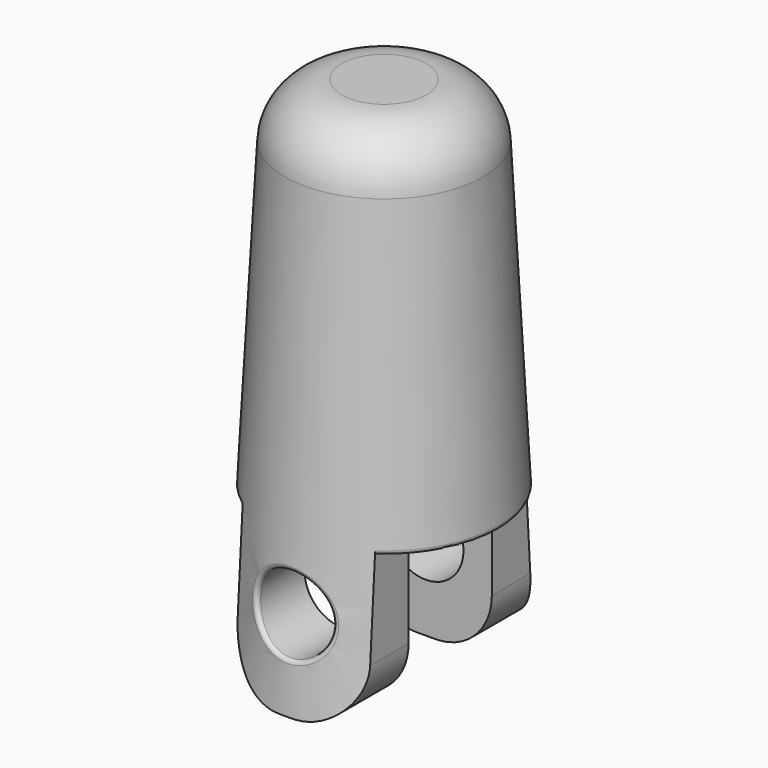
from build123d import *

# Parameters (mm, degrees)
F0_R          = 6.5
F1_DEPTH      = 27
F1_TAPER      = 3
F2_R          = 3
F3_W          = 1.5
F3_H          = 5.5
F3_W_2        = 7
F4_DEPTH      = 8
F5_R          = 2
F6_DEPTH      = 25
F6_DEPTH_BACK = 25
F7_T          = 1
F8_R          = 0.2
F9_R          = 3


# Not quite as in the source:
# - a shell that OpenCascade refuses in one call is made with other operations: the cavity is built on its own and cut out


with BuildPart() as f1:
    # F0 (on Top) → F1 (new body)
    with BuildSketch(Plane.XY):
        Circle(F0_R)
    extrude(amount=F1_DEPTH, taper=F1_TAPER)

    # F2
    f2_edges = [f1.edges().sort_by_distance(p)[0] for p in [
        (-5.08499, 0, 27),
    ]]
    fillet(f2_edges, radius=F2_R)

    # F3 (on Top) → F4 (cut)
    with BuildSketch(Plane.XY):
        Polygon((5, 2.75), (5, -2.75), (3.5, -2.75), (3.5, -6.25), (6.5, -6.25), (6.5, 6.25), (3.5, 6.25), (3.5, 2.75), align=None)
        with Locations((4.25, 0)):
            Rectangle(F3_W, F3_H)
        Rectangle(F3_W_2, F3_H)
        Polygon((-3.5, -6.25), (-3.5, -2.75), (-5, -2.75), (-5, 2.75), (-3.5, 2.75), (-3.5, 6.25), (-6.5, 6.25), (-6.5, -6.25), align=None)
        with Locations((-4.25, 0)):
            Rectangle(F3_W, F3_H)
    extrude(amount=F4_DEPTH, mode=Mode.SUBTRACT)

    # F5 (on face) → F6 (cut, two sides)
    with BuildSketch(Plane(origin=(0, -2.75, 0), x_dir=(-1, 0, 0), z_dir=(0, 1, 0))) as f6_sk:
        with Locations((0, 4.5984359458)):
            Circle(F5_R)
    extrude(amount=F6_DEPTH, mode=Mode.SUBTRACT)
    extrude(f6_sk.sketch, amount=-F6_DEPTH_BACK, mode=Mode.SUBTRACT)

    # F7: shell of thickness 1, made by hand


with BuildPart() as f7_core1:
    # F7_t2: copy of F1
    add(f1.part)

    # the walls: a layer under each face that stays
    f7_faces = [f7_core1.faces().sort_by_distance(p)[0] for p in [
        (-5.8669924317, 0, 12.0785039344),
        (3.5, -4.1136127875, 4),
        (0, -4.625, 0),
        (-3.5, -4.1136127875, 4),
        (-3.5, 4.1136127875, 4),
        (0, 4.625, 0),
        (3.5, 4.1136127875, 4),
        (-4.3031599863, 0, 26.176123113),
        (2, 4.5569343282, 4.5984359458),
        (2, -4.5569343282, 4.5984359458),
        (-2.3333333333, -2.75, 6.6666666667),
        (2.3333333333, 2.75, 6.6666666667),
        (0, 0, 27),
    ]]
    thicken(f7_faces, amount=-F7_T, mode=Mode.SUBTRACT)


with BuildPart() as f1_1:
    add(f1.part)

    # what is left inside the walls is the cavity
    f7_cavity = [f7_core1.part.solids().sort_by_distance(p)[0] for p in [
        (0, -4.859979, 1.588436),
        (-4.848949, 0, 12.205533),
        (0, 4.859979, 1.588436),
    ]]
    add(f7_cavity, mode=Mode.SUBTRACT)

    # F8
    f8_edges = [f1_1.edges().sort_by_distance(p)[0] for p in [
        (1.999873, -5.932154, 4.575894),
        (5.397127, -2.801142, 8),
        (-6.080738, 0, 8),
        (5.397127, 2.801142, 8),
        (1.999882, 5.932105, 4.576739),
    ]]
    fillet(f8_edges, radius=F8_R)

    # F9
    f9_edges = [f1_1.edges().sort_by_distance(p)[0] for p in [
        (3.5, -4.113613, 0),
        (3.5, 4.113613, 0),
        (-3.5, 4.113613, 0),
        (-3.5, -4.113613, 0),
    ]]
    fillet(f9_edges, radius=F9_R)


solid = f1_1.part
